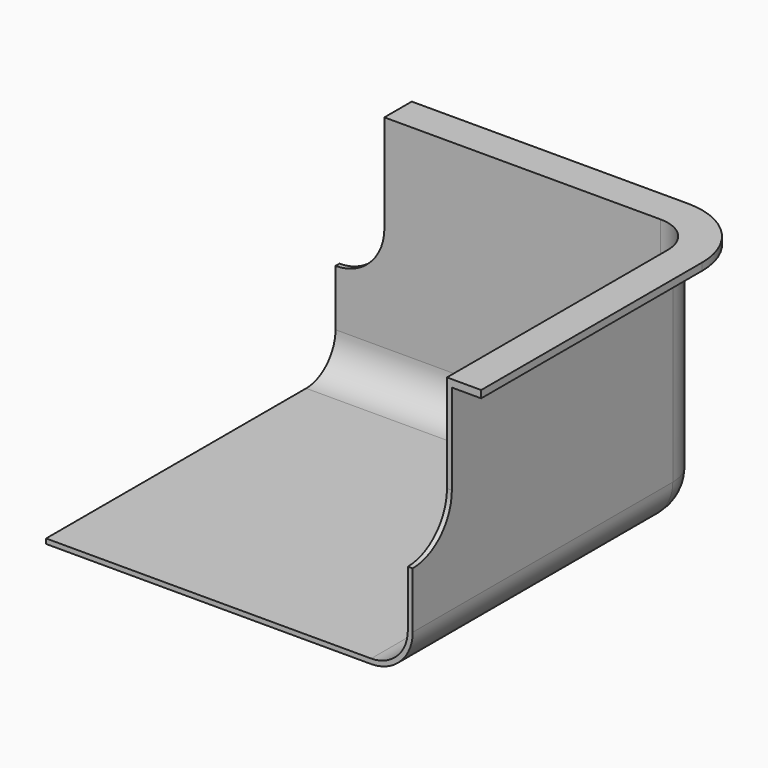
from build123d import *

# Parameters (mm, degrees)
F1_DEPTH  = 100
F2_W      = 150
F2_H      = 150
F3_DEPTH  = 2
F4_R      = 15
F5_R      = 17
F7_DEPTH  = 150.001
F10_DEPTH = 3


# Not quite as in the source:
# - a pattern or mirror of a feature is missing from the dataset's text; its kind, count and spacing are read off the source's solid


with BuildPart() as f1:
    # F0 (on Top) → F1 (new body)
    with BuildSketch(Plane.XY):
        Polygon((0, 0), (-150, 0), (-150, -2), (-2, -2), (-2, -150), (0, -150), align=None)
    extrude(amount=F1_DEPTH)

    # F2 (on face) → F3 (join)
    with BuildSketch(Plane(origin=(0, 0, 0), x_dir=(1, 0, 0), z_dir=(0, 0, -1))):
        with Locations((-75, 75)):
            Rectangle(F2_W, F2_H)
    extrude(amount=-F3_DEPTH)

    # F4
    f4_edges = [f1.edges().sort_by_distance(p)[0] for p in [
        (-2, -76, 2),
        (-76, -2, 2),
        (-2, -2, 51),
    ]]
    fillet(f4_edges, radius=F4_R)

    # F5
    f5_edges = [f1.edges().sort_by_distance(p)[0] for p in [
        (0, -75, 0),
        (-75, 0, 0),
        (0, 0, 50),
    ]]
    fillet(f5_edges, radius=F5_R)

    # F6 (on face) → F7 (cut, through all)
    with BuildSketch(Plane.YZ):
        with BuildLine():
            Line((-150, 100), (-150, 40))
            ThreePointArc((-150, 40), (-135.8578643763, 45.8578643763), (-130, 60))
            Line((-130, 60), (-130, 100))
            Line((-130, 100), (-150, 100))
        make_face()
    f7 = extrude(amount=-F7_DEPTH, mode=Mode.SUBTRACT)

    # F7_copies: F7 across plane
    add(f7.mirror(Plane(origin=(0, 0, 0), x_dir=(-0.7071067812, -0.7071067812, 0), z_dir=(-0.7071067812, 0.7071067812, 0))), mode=Mode.SUBTRACT)

    # F9 (on face) → F10 (join)
    with BuildSketch(Plane.XY.offset(100)):
        with BuildLine():
            Line((-130, 12), (-130, 0))
            Line((-130, 0), (-17, 0))
            ThreePointArc((-17, 0), (-4.9791847198, -4.9791847198), (0, -17))
            Line((0, -17), (0, -130))
            Line((0, -130), (12, -130))
            Line((12, -130), (12, -17))
            ThreePointArc((12, -17), (3.5060966544, 3.5060966544), (-17, 12))
            Line((-17, 12), (-130, 12))
        make_face()
    extrude(amount=-F10_DEPTH)


solid = f1.part
